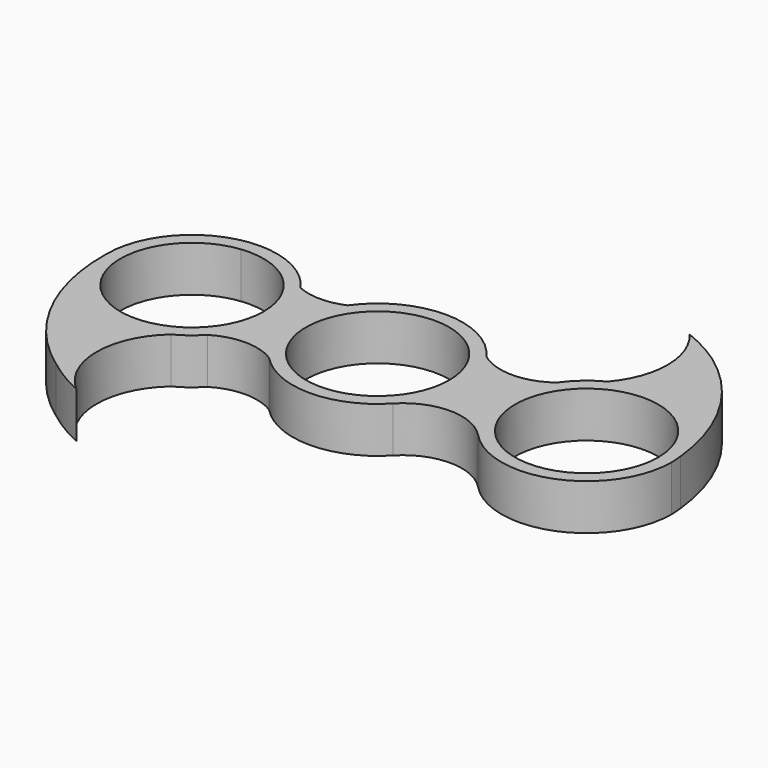
from build123d import *

# Parameters (mm, degrees)
F0_R     = 10.95
F1_DEPTH = 7


# Not quite as in the source:
# - a feature names something its author has since deleted; it is built from what else it names


with BuildPart() as f1:
    # F0 (on Top) → F1 (new body)
    with BuildSketch(Plane.XY):
        with BuildLine():
            ThreePointArc((-20.552952936, -6.752012725), (-17.9358713071, -2.6350535567), (-17.0205455745, 2.1566734649))
            ThreePointArc((-17.0205455745, 2.1566734649), (-17.6332758432, 6.1007257723), (-19.4137068981, 9.672987275))
            ThreePointArc((-19.4137068981, 9.672987275), (-33.9645978819, 14.5439431963), (-43.0205455745, 2.1566734649))
            ThreePointArc((-43.0205455745, 2.1566734649), (-36.7659143561, -8.9563819205), (-24.0205455745, -9.3758891297))
            ThreePointArc((-24.0205455745, -9.3758891297), (-22.176261837, -8.2099659445), (-20.552952936, -6.752012725))
        make_face()
        with BuildLine():
            ThreePointArc((-31.2069165924, 13.042215427), (-22.7091935329, 10.3081537797), (-19.0705455745, 2.1566734649))
            ThreePointArc((-19.0705455745, 2.1566734649), (-22.7091935329, -5.9948068499), (-31.2069165924, -8.7288684971))
            ThreePointArc((-31.2069165924, -8.7288684971), (-40.9705455745, 2.1566734649), (-31.2069165924, 13.042215427))
        make_face(mode=Mode.SUBTRACT)
        with BuildLine():
            ThreePointArc((-19.4137068981, 9.672987275), (-17.6332758432, 6.1007257723), (-17.0205455745, 2.1566734649))
            ThreePointArc((-17.0205455745, 2.1566734649), (-17.9358713071, -2.6350535567), (-20.552952936, -6.752012725))
            ThreePointArc((-20.552952936, -6.752012725), (-15.8304691356, -5.4134843039), (-11.1079853352, -6.752012725))
            ThreePointArc((-11.1079853352, -6.752012725), (-14.6092343722, 1.2571482598), (-12.2472313731, 9.672987275))
            ThreePointArc((-12.2472313731, 9.672987275), (-15.8304691356, 8.9289189085), (-19.4137068981, 9.672987275))
        make_face()
        with BuildLine():
            ThreePointArc((-24.0205455745, -9.3758891297), (-36.7659143561, -8.9563819205), (-43.0205455745, 2.1566734649))
            ThreePointArc((-43.0205455745, 2.1566734649), (-39.7569738909, -12.4615406932), (-30.0205455745, -23.8433265351))
            ThreePointArc((-30.0205455745, -23.8433265351), (-27.1231782319, -25.8236586783), (-24.0205455745, -27.4638182769))
            ThreePointArc((-24.0205455745, -27.4638182769), (-28.1334228551, -18.4198537033), (-24.0205455745, -9.3758891297))
        make_face()
        with BuildLine():
            ThreePointArc((8.9664459798, 9.672987275), (-1.6403926966, 15.1566734649), (-12.2472313731, 9.672987275))
            ThreePointArc((-12.2472313731, 9.672987275), (-14.6092343722, 1.2571482598), (-11.1079853352, -6.752012725))
            ThreePointArc((-11.1079853352, -6.752012725), (-1.6403926966, -10.8433265351), (7.8271999419, -6.752012725))
            ThreePointArc((7.8271999419, -6.752012725), (10.4442815708, -2.6350535567), (11.3596073034, 2.1566734649))
            ThreePointArc((11.3596073034, 2.1566734649), (10.7468770347, 6.1007257723), (8.9664459798, 9.672987275))
        make_face()
        with Locations((-1.6403926966, 2.1566734649)):
            Circle(F0_R, mode=Mode.SUBTRACT)
        with BuildLine():
            ThreePointArc((19.7036979596, 9.672987275), (14.3350719697, 7.8964113233), (8.9664459798, 9.672987275))
            ThreePointArc((8.9664459798, 9.672987275), (10.7468770347, 6.1007257723), (11.3596073034, 2.1566734649))
            ThreePointArc((11.3596073034, 2.1566734649), (10.4442815708, -2.6350535567), (7.8271999419, -6.752012725))
            ThreePointArc((7.8271999419, -6.752012725), (14.3350719697, -3.9687322514), (20.8429439975, -6.752012725))
            ThreePointArc((20.8429439975, -6.752012725), (17.3416949605, 1.2571482598), (19.7036979596, 9.672987275))
        make_face()
        with BuildLine():
            ThreePointArc((24.310536636, 13.6892360596), (21.767742229, 11.9556868703), (19.7036979596, 9.672987275))
            ThreePointArc((19.7036979596, 9.672987275), (17.3416949605, 1.2571482598), (20.8429439975, -6.752012725))
            ThreePointArc((20.8429439975, -6.752012725), (35.1022636576, -9.9280008025), (43.310536636, 2.1566734649))
            ThreePointArc((43.310536636, 2.1566734649), (43.2572345725, 3.0913245901), (43.1757344795, 4.0239400363))
            ThreePointArc((43.1757344795, 4.0239400363), (36.2382024635, 13.7265817549), (24.310536636, 13.6892360596))
        make_face()
        with Locations((30.310536636, 2.1566734649)):
            Circle(F0_R, mode=Mode.SUBTRACT)
        with BuildLine():
            ThreePointArc((24.310536636, 29.3296992304), (27.2086699071, 21.509467645), (24.310536636, 13.6892360596))
            ThreePointArc((24.310536636, 13.6892360596), (36.2382024635, 13.7265817549), (43.1757344795, 4.0239400363))
            ThreePointArc((43.1757344795, 4.0239400363), (39.126790521, 16.45868474), (30.310536636, 26.1173849869))
            ThreePointArc((30.310536636, 26.1173849869), (27.3989585648, 27.8886976733), (24.310536636, 29.3296992304))
        make_face()
    extrude(amount=F1_DEPTH)


solid = f1.part
